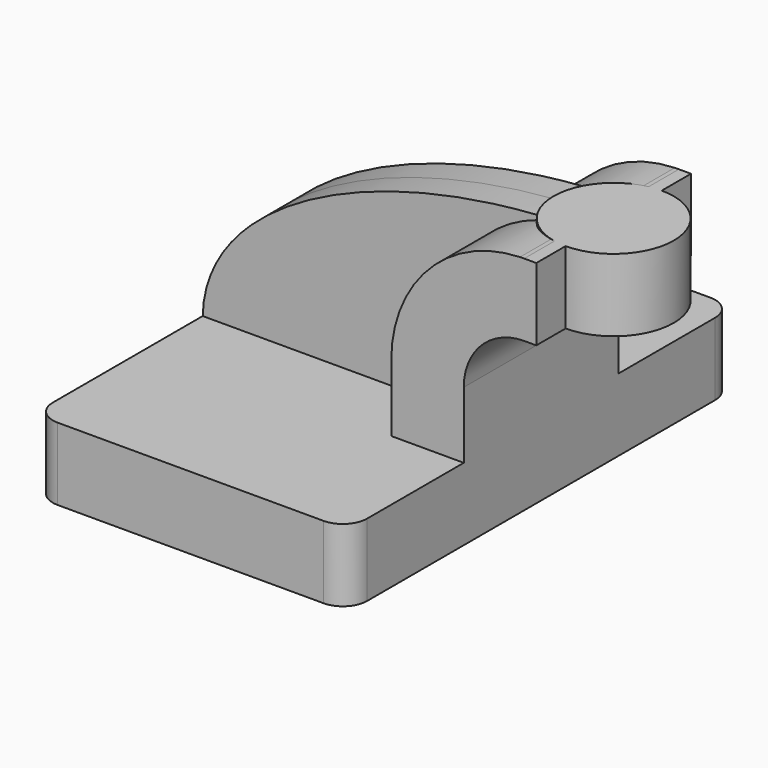
from build123d import *

# Parameters (mm, degrees)
F1_DEPTH = 63.5
F2_DEPTH = 25.4
F3_DEPTH = 7.9375
F0_W     = 15.7855516109
F0_H     = 19.05
F5_R     = 6.35


with BuildPart() as f1:
    # F0 (on Front) → F1 (new body, symmetric)
    with BuildSketch(Plane.XZ):
        Polygon((-41.275, 9.525), (-41.275, -9.525), (41.275, -9.525), (41.275, 9.525), (22.225, 9.525), align=None)
    extrude(amount=F1_DEPTH, both=True)

    # F0 (on Front) → F2 (join, symmetric)
    with BuildSketch(Plane.XZ):
        with BuildLine():
            Line((22.225, 9.525), (41.275, 9.525))
            Line((41.275, 9.525), (41.275, 27.0002))
            ThreePointArc((41.275, 27.0002), (45.9246798487, 38.2255201513), (57.15, 42.8752))
            Line((57.15, 42.8752), (60.325, 42.8752))
            Line((60.325, 42.8752), (60.325, 61.9252))
            Line((60.325, 61.9252), (57.15, 61.9252))
            add(Edge.make_bspline(
                [(56.0507958514, 61.9078979367), (56.4168804985, 61.9147360597), (56.7832864431, 61.9205050971), (57.15, 61.9252)],
                knots=[110.7182330401, 110.7182330401, 110.7182330401, 110.7182330401, 111.5045361635, 111.5045361635, 111.5045361635, 111.5045361635], degree=3))
            ThreePointArc((56.0507958514, 61.9078979367), (32.0686789633, 51.3041700472), (22.225, 27.0002))
            Line((22.225, 27.0002), (22.225, 9.525))
        make_face()
    extrude(amount=F2_DEPTH, both=True)

    # F0 (on Front) → F3 (join, symmetric)
    with BuildSketch(Plane.XZ):
        with BuildLine():
            add(Edge.make_bspline(
                [(-41.275, 9.525), (-40.6745437573, 38.785344003), (4.5029333836, 60.945031492), (56.0507958514, 61.9078979367)],
                knots=[0, 0, 0, 0, 110.7182330401, 110.7182330401, 110.7182330401, 110.7182330401], degree=3))
            Line((-41.275, 9.525), (22.225, 9.525))
            Line((22.225, 9.525), (22.225, 27.0002))
            ThreePointArc((22.225, 27.0002), (32.0686789633, 51.3041700472), (56.0507958514, 61.9078979367))
        make_face()
    extrude(amount=F3_DEPTH, both=True)

    # F0 (on Front) → F4 (revolve)
    with BuildSketch(Plane.XZ):
        with Locations((68.2177758054, 52.4002)):
            Rectangle(F0_W, F0_H)
    revolve(axis=Axis((60.325, 0, 52.3875), (0, 0, 1)))

    # F5
    f5_edges = [f1.edges().sort_by_distance(p)[0] for p in [
        (41.275, -63.5, 0),
        (-41.275, -63.5, 0),
        (41.275, 63.5, 0),
        (-41.275, 63.5, 0),
    ]]
    fillet(f5_edges, radius=F5_R)


solid = f1.part
